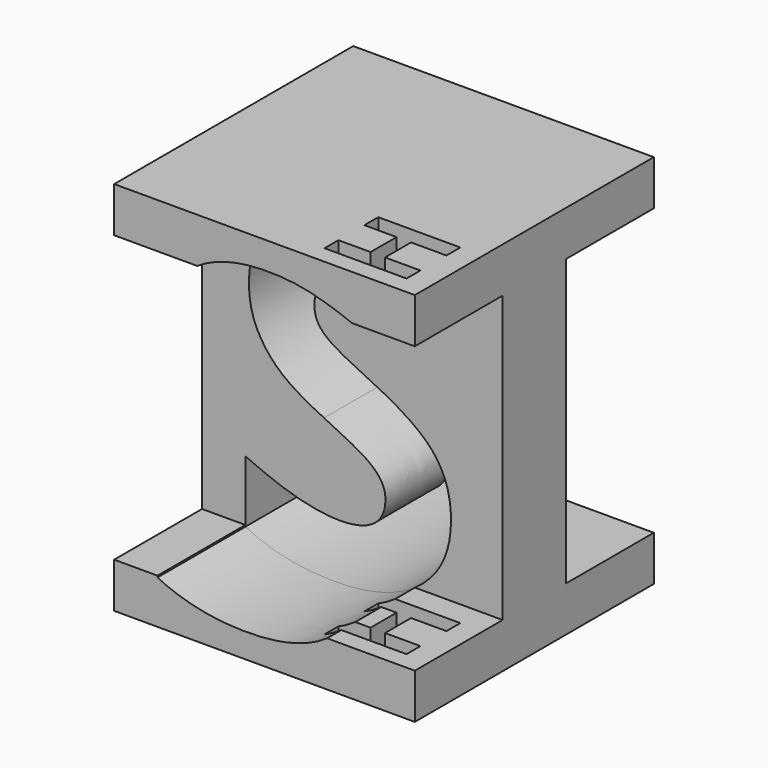
from build123d import *

# Parameters (mm, degrees)
F0_W          = 25.4
F0_H          = 31.75
F1_DEPTH      = 31.75
F3_DEPTH      = 25.401
F4_TEXT_SIZE  = 37.3493263415
F5_DEPTH      = 15.9659485267
F5_DEPTH_BACK = 9.2802512261
F6_TEXT_SIZE  = 9.7093582947
F7_DEPTH      = 27.9410001
F7_DEPTH_BACK = 3.8110001


# Not quite as in the source:
# - Text() gives the source's letters only with a copy of the font that has no kerning and outlines rounded to 1/6400 em; it was checked with that copy


with BuildPart() as f1:
    # F0 (on Front) → F1 (new body)
    with BuildSketch(Plane.XZ):
        Rectangle(F0_W, F0_H)
    extrude(amount=F1_DEPTH)

    # F2 (on face) → F3 (cut, through all)
    with BuildSketch(Plane(origin=(-12.7, 0, 0), x_dir=(0, -1, 0), z_dir=(-1, 0, 0))):
        Polygon((28.4970998764, -12.065), (28.4970998764, -15.875), (31.75, -15.875), (31.75, 15.875), (28.4970998764, 15.875), (28.4970998764, 12.065), (19.2178486503, 12.065), (19.2178486503, -12.065), align=None)
        Polygon((0, -15.875), (3.2529001236, -15.875), (3.2529001236, -12.065), (12.5412535983, -12.065), (12.5412535983, 12.065), (3.2529001236, 12.065), (3.2529001236, 15.875), (0, 15.875), align=None)
    extrude(amount=-F3_DEPTH, mode=Mode.SUBTRACT)

    # F4 (on face) → F5 (cut, two sides)
    with BuildSketch(Plane.XZ.offset(19.2178486503)) as f5_sk:
        with Locations((-10.758356736, -13.4457574829)):
            Text('S', F4_TEXT_SIZE, font='Open Sans', font_style=FontStyle.BOLD, text_align=(TextAlign.LEFT, TextAlign.BOTTOM))
    extrude(amount=-F5_DEPTH, mode=Mode.SUBTRACT)
    extrude(f5_sk.sketch, amount=F5_DEPTH_BACK, mode=Mode.SUBTRACT)

    # F6 (on face) → F7 (cut, two sides)
    with BuildSketch(Plane.XY.offset(-12.065)) as f7_sk:
        with Locations(Location((10.795, -27.8620998764), (0, 0, 90))):
            Text('H', F6_TEXT_SIZE, font='Open Sans', font_style=FontStyle.BOLD, text_align=(TextAlign.LEFT, TextAlign.BOTTOM))
    extrude(amount=F7_DEPTH, mode=Mode.SUBTRACT)
    extrude(f7_sk.sketch, amount=-F7_DEPTH_BACK, mode=Mode.SUBTRACT)


solid = f1.part
